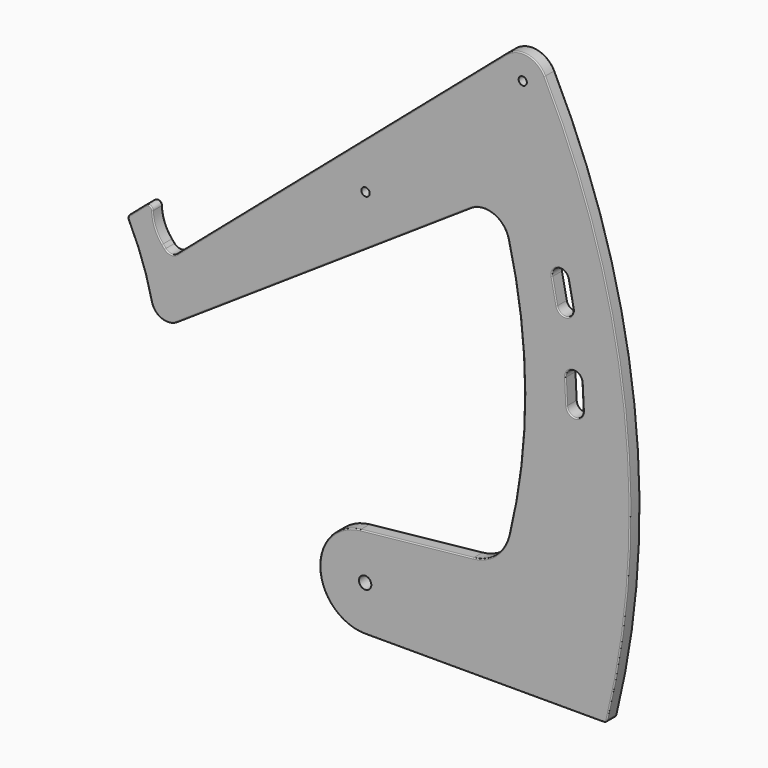
from build123d import *

# Parameters (mm, degrees)
F1_DEPTH = 6
F3_DEPTH = 6.001
F4_R     = 12
F5_R     = 8
F6_R     = 4
F7_R     = 20
F8_R     = 12
F10_D    = 6
F12_D    = 4
F13_R    = 2
F14_R    = 0.5


# Not quite as in the source:
# - a feature names something its author has since deleted; it is built from what else it names


with BuildPart() as f1:
    # F0 (on Front) → F1 (new body)
    with BuildSketch(Plane.XZ):
        with BuildLine():
            ThreePointArc((102.7003738081, 43.8794816981), (83.0301502354, 20.8486089627), (105, 0))
            Line((105, 0), (222, 0))
            ThreePointArc((222, 0), (230.2673095695, 143.5371087645), (185, 280))
            Line((185, 280), (10.6440422584, 130))
            Line((10.6440422584, 130), (6.7309987801, 134.5484162889))
            ThreePointArc((6.7309987801, 134.5484162889), (2.4989452542, 142.7084609792), (2.3663393595, 151.8997080148))
            Line((2.3663393595, 151.8997080148), (-10.5208401257, 140.812751493))
            ThreePointArc((-10.5208401257, 140.812751493), (-1.6535359727, 119.2796291851), (3.3812292532, 96.5429720343))
            Line((3.3812292532, 96.5429720343), (169.761000021, 207.5284299973))
            ThreePointArc((169.761000021, 207.5284299973), (182.3801238188, 129.3882640434), (171, 51.0580616779))
            Line((171, 51.0580616779), (102.7003738081, 43.8794816981))
        make_face()
    extrude(amount=F1_DEPTH)

    # F2 (on Front) → F3 (cut, through all)
    with BuildSketch(Plane.XZ):
        with BuildLine():
            ThreePointArc((203.5177584626, 183.6778955659), (198.811812282, 186.817014956), (195.6726928919, 182.1110687753))
            Line((195.6726928919, 182.1110687753), (198.0229330778, 170.3434704193))
            ThreePointArc((198.0229330778, 170.3434704193), (202.7288792584, 167.2043510293), (205.8679986485, 171.9102972099))
            Line((205.8679986485, 171.9102972099), (203.5177584626, 183.6778955659))
        make_face()
        with BuildLine():
            ThreePointArc((210.2223788251, 141.6319319116), (206.0293672683, 145.4291221998), (202.2321769801, 141.236110643))
            Line((202.2321769801, 141.236110643), (202.825908883, 129.2508078755))
            ThreePointArc((202.825908883, 129.2508078755), (207.0189204398, 125.4536175874), (210.816110728, 129.6466291441))
            Line((210.816110728, 129.6466291441), (210.2223788251, 141.6319319116))
        make_face()
    extrude(amount=F3_DEPTH, mode=Mode.SUBTRACT)

    # F4
    f4_edges = [f1.edges().sort_by_distance(p)[0] for p in [
        (185, -3, 280),
    ]]
    fillet(f4_edges, radius=F4_R)

    # F5
    f5_edges = [f1.edges().sort_by_distance(p)[0] for p in [
        (3.381229, -3, 96.542972),
    ]]
    fillet(f5_edges, radius=F5_R)

    # F6
    f6_edges = [f1.edges().sort_by_distance(p)[0] for p in [
        (10.644042, -3, 130),
    ]]
    fillet(f6_edges, radius=F6_R)

    # F7
    f7_edges = [f1.edges().sort_by_distance(p)[0] for p in [
        (171, -3, 51.058062),
    ]]
    fillet(f7_edges, radius=F7_R)

    # F8
    f8_edges = [f1.edges().sort_by_distance(p)[0] for p in [
        (169.761, -3, 207.52843),
    ]]
    fillet(f8_edges, radius=F8_R)

    # F10 (through all)
    with Locations(Plane(origin=(0, 0, 0), x_dir=(1, 0, 0), z_dir=(0, 1, 0))):
        with Locations((105, -22)):
            Hole(F10_D / 2)

    # F12 (through all)
    with Locations(Plane(origin=(0, 0, 0), x_dir=(1, 0, 0), z_dir=(0, 1, 0))):
        with Locations((105.212829657, -188.9329911228), (181.4589475746, -261.1239150848)):
            Hole(F12_D / 2)

    # F13
    f13_edges = [f1.edges().sort_by_distance(p)[0] for p in [
        (-10.52084, -3, 140.812751),
        (2.366339, -3, 151.899708),
        (222, -3, 0),
    ]]
    fillet(f13_edges, radius=F13_R)

    # F14
    f14_edges = [f1.edges().sort_by_distance(p)[0] for p in [
        (93.65459, -6, 201.414722),
        (130.073752, 0, 46.75654),
        (-3.294044, -6, 124.174238),
        (84.833006, -6, 150.876276),
        (84.833006, 0, 150.876276),
        (-3.294044, 0, 124.174238),
        (-9.986863, 0, 140.713386),
        (6.135602, 0, 102.558545),
        (-5.367429, 0, 145.246278),
        (0.715162, 0, 148.965378),
        (167.080901, 0, 199.641106),
        (3.21438, 0, 140.443038),
        (182.387204, 0, 128.08015),
        (7.383173, 0, 133.790347),
        (168.494422, 0, 54.444361),
        (10.768107, 0, 131.652203),
        (93.65459, 0, 201.414722),
        (83.03015, 0, 20.848609),
        (183.789671, 0, 272.895395),
        (162.718762, 0, 0),
        (231.102181, 0, 136.753387),
        (221.670414, 0, 0.425204),
        (-9.986863, -6, 140.713386),
        (6.135602, -6, 102.558545),
        (-5.367429, -6, 145.246278),
        (0.715162, -6, 148.965378),
        (167.080901, -6, 199.641106),
        (3.21438, -6, 140.443038),
        (182.387204, -6, 128.08015),
        (7.383173, -6, 133.790347),
        (168.494422, -6, 54.444361),
        (10.768107, -6, 131.652203),
        (130.073752, -6, 46.75654),
        (83.03015, -6, 20.848609),
        (183.789671, -6, 272.895395),
        (162.718762, -6, 0),
        (231.102181, -6, 136.753387),
        (221.670414, -6, 0.425204),
        (210.519245, -6, 135.639281),
        (207.01892, -6, 125.453618),
        (206.029367, -6, 145.429122),
        (202.529043, -6, 135.243459),
        (202.728879, -6, 167.204351),
        (196.847813, -6, 176.22727),
        (204.692879, -6, 177.794096),
        (198.811812, -6, 186.817015),
    ]]
    fillet(f14_edges, radius=F14_R)


solid = f1.part
